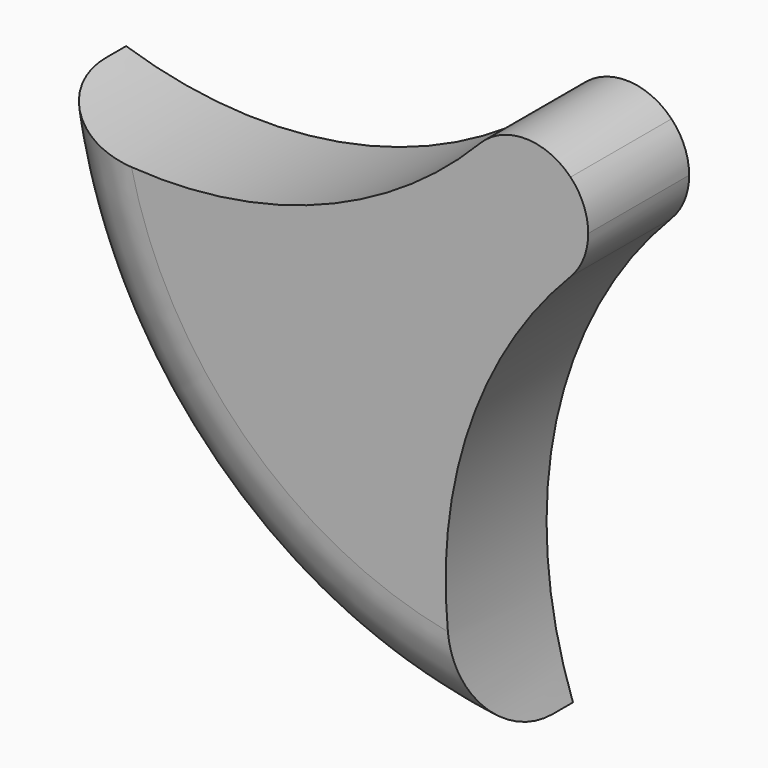
from build123d import *

# Parameters (mm, degrees)
F1_DEPTH = 6.35
F2_R     = 5.08


with BuildPart() as f1:
    # F0 (on Front) → F1 (new body)
    with BuildSketch(Plane.XZ):
        with BuildLine():
            ThreePointArc((-25.1582770203, -3.4958686142), (-17.6652781796, -18.2509711204), (-2.6737065925, -25.2588854279))
            ThreePointArc((-2.6737065925, -25.2588854279), (-3.505224173, -13.0246794199), (2.277990057, -2.2116478698))
            ThreePointArc((2.277990057, -2.2116478698), (-2.2081596575, -2.2813715013), (-2.2847476043, 2.2046662752))
            ThreePointArc((-2.2847476043, 2.2046662752), (-12.90346397, -3.9280392538), (-25.1582770203, -3.4958686142))
        make_face()
        with BuildLine():
            ThreePointArc((-2.2847476043, 2.2046662752), (-2.2081596575, -2.2813715013), (2.277990057, -2.2116478698))
            ThreePointArc((2.277990057, -2.2116478698), (2.942213744, -1.1933160874), (3.175, 0))
            ThreePointArc((3.175, 0), (2.9440362131, 1.1888127589), (2.2847475428, 2.2046663389))
            ThreePointArc((2.2847475428, 2.2046663389), (-4.43e-08, 3.175), (-2.2847476043, 2.2046662752))
        make_face()
    extrude(amount=F1_DEPTH)

    # F2
    f2_edges = [f1.edges().sort_by_distance(p)[0] for p in [
        (-17.665278, -6.35, -18.250971),
    ]]
    fillet(f2_edges, radius=F2_R)


solid = f1.part
